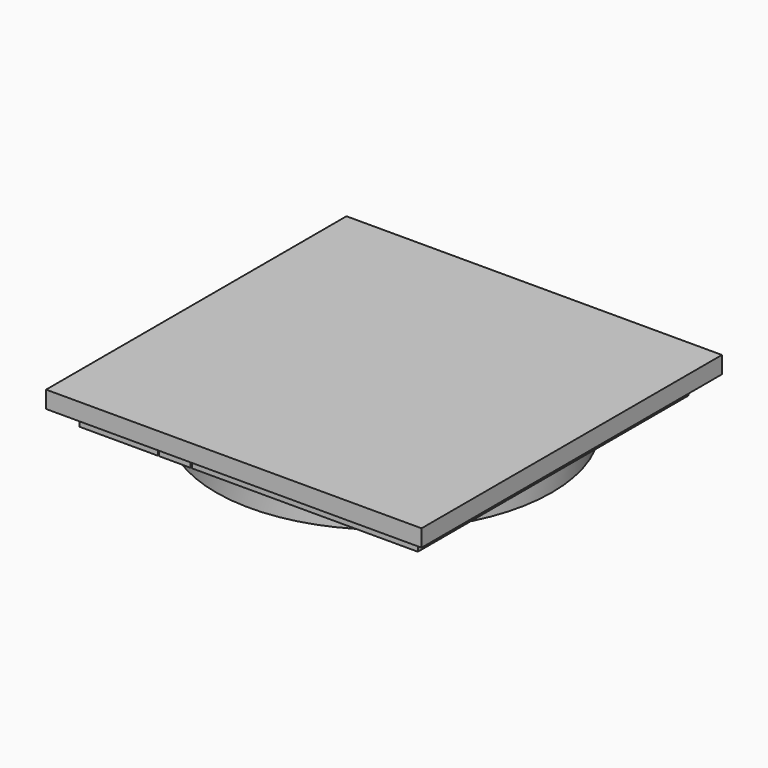
from build123d import *

# Parameters (mm, degrees)
F2_R           = 2.5
F4_DEPTH       = 5
F5_START       = 5
F3_W           = 110
F3_H           = 110
F3_W_2         = 100
F3_H_2         = 100
F5_DEPTH       = 5
F2_W           = 9.2
F2_H           = 32.6
F6_DEPTH       = 5
F8_R           = 49.2
F9_DEPTH       = 5
F10_COUNT      = 4
F11_D          = 5
F12_D          = 5
F15_DEPTH      = 5
F16_DEPTH      = 15
F16_DEPTH_BACK = 5


# Not quite as in the source:
# - a feature names something its author has since deleted; it is built from what else it names


with BuildPart() as f4:
    # F2 (on Top) → F4 (new body)
    with BuildSketch(Plane.XY):
        Polygon((-49.6, 49.6), (-49.6, 26.6), (-16.6, 26.6), (-16.6, 16.6), (-49.6, 16.6), (-49.6, -49.6), (-26.6, -49.6), (-26.6, -16.6), (-16.6, -16.6), (-16.6, -49.6), (49.6, -49.6), (49.6, -26.6), (16.6, -26.6), (16.6, -16.6), (49.6, -16.6), (49.6, 49.6), (26.6, 49.6), (26.6, 16.6), (16.6, 16.6), (16.6, 49.6), align=None)
        Circle(F2_R, mode=Mode.SUBTRACT)
    extrude(amount=F4_DEPTH)

    # F3 (on Top) → F5 (join)
    with BuildSketch(Plane.XY.offset(F5_START)):
        Rectangle(F3_W, F3_H)
        Rectangle(F3_W_2, F3_H_2, mode=Mode.SUBTRACT)
        Rectangle(F3_W_2, F3_H_2)
    extrude(amount=F5_DEPTH)


with BuildPart() as f6:
    # F2 (on Top) → F6 (new body)
    with BuildSketch(Plane.XY):
        with Locations((21.6, 33.3)):
            Rectangle(F2_W, F2_H)
    extrude(amount=F6_DEPTH)


with BuildPart() as f9:
    # F8 (on Top) → F9 (new body)
    with BuildSketch(Plane.XY):
        Circle(F8_R)
    extrude(amount=-F9_DEPTH)

    # F12 (through all)
    with Locations(Plane.XY):
        with Locations((0, 0)):
            Hole(F12_D / 2)

    # F14 (on Top) → F15 (cut, through all)
    with BuildSketch(Plane.XY):
        with BuildLine():
            ThreePointArc((-20.3400950888, 19.2442236945), (-18.9604427499, 22.5761239667), (-22.2923430221, 23.9557763055))
            ThreePointArc((-22.2923430221, 23.9557763055), (-33.9277402962, 14.4051091441), (-38.2970129473, 0))
            ThreePointArc((-38.2970129473, 0), (-35.7470129473, -2.55), (-33.1970129473, 0))
            ThreePointArc((-33.1970129473, 0), (-29.6870761701, 11.571954053), (-20.3400950888, 19.2442236945))
        make_face()
        with BuildLine():
            ThreePointArc((-19.2442236945, -20.3400950888), (-22.5761239667, -18.9604427499), (-23.9557763055, -22.2923430221))
            ThreePointArc((-23.9557763055, -22.2923430221), (-14.4051091441, -33.9277402962), (0, -38.2970129473))
            ThreePointArc((0, -38.2970129473), (2.55, -35.7470129473), (0, -33.1970129473))
            ThreePointArc((0, -33.1970129473), (-11.571954053, -29.6870761701), (-19.2442236945, -20.3400950888))
        make_face()
        with BuildLine():
            ThreePointArc((20.3400950888, -19.2442236945), (18.9604427499, -22.5761239667), (22.2923430221, -23.9557763055))
            ThreePointArc((22.2923430221, -23.9557763055), (33.9277402962, -14.4051091441), (38.2970129473, 0))
            ThreePointArc((38.2970129473, 0), (35.7470129473, 2.55), (33.1970129473, 0))
            ThreePointArc((33.1970129473, 0), (29.6870761701, -11.571954053), (20.3400950888, -19.2442236945))
        make_face()
        with BuildLine():
            ThreePointArc((19.2442236945, 20.3400950888), (22.5761239667, 18.9604427499), (23.9557763055, 22.2923430221))
            ThreePointArc((23.9557763055, 22.2923430221), (14.4051091441, 33.9277402962), (0, 38.2970129473))
            ThreePointArc((0, 38.2970129473), (-2.55, 35.7470129473), (0, 33.1970129473))
            ThreePointArc((0, 33.1970129473), (11.571954053, 29.6870761701), (19.2442236945, 20.3400950888))
        make_face()
    extrude(amount=-F15_DEPTH, mode=Mode.SUBTRACT)


with BuildPart() as f10_1:
    # F10: instance of F6
    add(f6.part.rotate(Axis((0, 0, 5), (0, 0, 1)), 1 * 360 / F10_COUNT))


with BuildPart() as f10_2:
    # F10: instance of F6
    add(f6.part.rotate(Axis((0, 0, 5), (0, 0, 1)), 2 * 360 / F10_COUNT))


with BuildPart() as f10_3:
    # F10: instance of F6
    add(f6.part.rotate(Axis((0, 0, 5), (0, 0, 1)), 3 * 360 / F10_COUNT))


with BuildPart() as f6_1:
    add(f6.part)

    # F11 (through all)
    with Locations(Plane(origin=(0, 0, 0), x_dir=(1, 0, 0), z_dir=(0, 0, -1))):
        with Locations((21.6, -21.6)):
            Hole(F11_D / 2)


with BuildPart() as f16:
    # F2 (on Top) → F16 (new body, two sides)
    with BuildSketch(Plane.XY) as f16_sk:
        Circle(F2_R)
    extrude(amount=-F16_DEPTH)
    extrude(f16_sk.sketch, amount=F16_DEPTH_BACK)


solid = Compound([f4.part, f9.part, f10_1.part, f10_2.part, f10_3.part, f6_1.part, f16.part])
